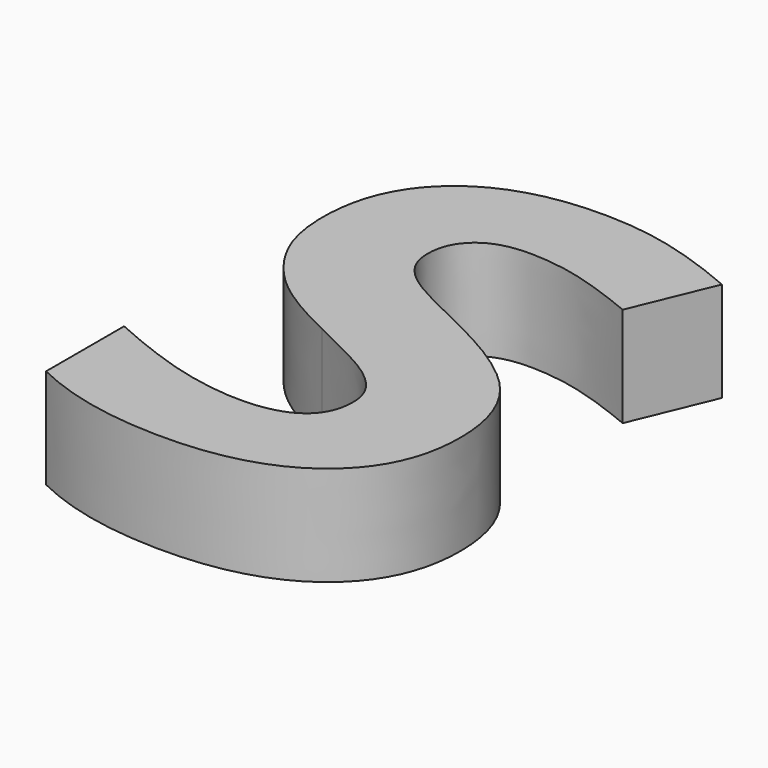
from build123d import *

# Parameters (mm, degrees)
F0_TEXT_SIZE = 6.9433143477
F1_DEPTH     = 1


# Not quite as in the source:
# - Text() gives the source's letters only with a copy of the font that has no kerning and outlines rounded to 1/6400 em; it was checked with that copy


with BuildPart() as f1:
    # F0 (on Top) → F1 (new body)
    with BuildSketch(Plane.XY):
        with Locations((-21.5482173689, -1.2928930377)):
            Text('S', F0_TEXT_SIZE, font='Open Sans', font_style=FontStyle.BOLD, text_align=(TextAlign.LEFT, TextAlign.BOTTOM))
    extrude(amount=F1_DEPTH)


solid = f1.part
